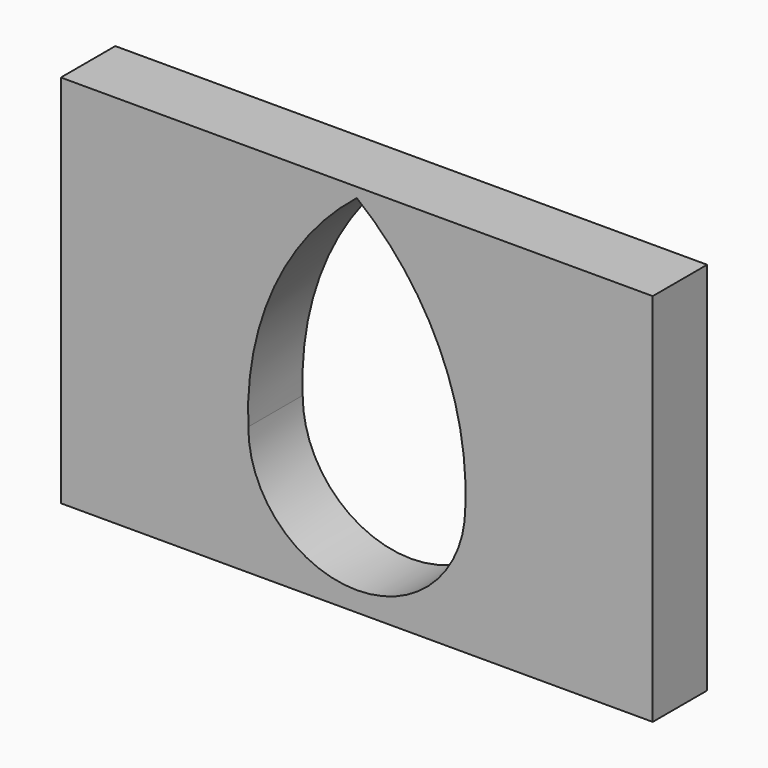
from build123d import *

# Parameters (mm, degrees)
F0_W     = 60
F0_H     = 6.8944109904
F1_DEPTH = 38
F3_DEPTH = 25


with BuildPart() as f1:
    # F0 (on Top) → F1 (new body)
    with BuildSketch(Plane.XY):
        with Locations((-5.1953140646, 10.8007821254)):
            Rectangle(F0_W, F0_H)
    extrude(amount=F1_DEPTH)

    # F2 (on face) → F3 (cut)
    with BuildSketch(Plane.XZ.offset(-7.3535766302)):
        with BuildLine():
            ThreePointArc((-5.1953140646, 37), (-13.5847741794, 26.3243358859), (-16.1953140646, 13))
            ThreePointArc((-16.1953140646, 13), (-5.1953140646, 2), (5.8046859354, 13))
            ThreePointArc((5.8046859354, 13), (3.1941460502, 26.3243358859), (-5.1953140646, 37))
        make_face()
    extrude(amount=-F3_DEPTH, mode=Mode.SUBTRACT)


solid = f1.part
